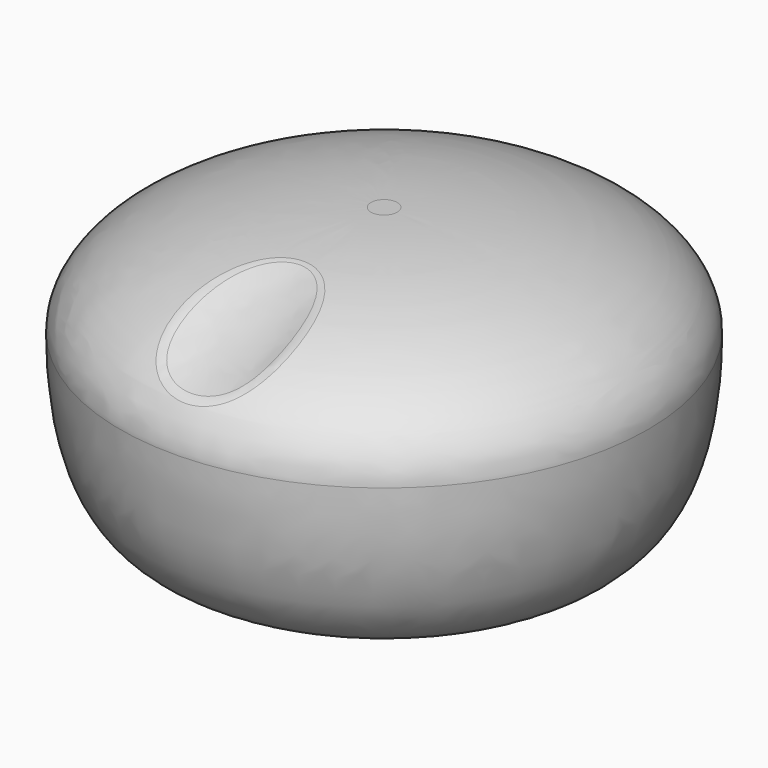
from build123d import *

# Parameters (mm, degrees)
F2_DEPTH  = 6.4135
F1_W      = 4.572
F1_H      = 1.397
F3_DEPTH  = 3.556
F5_W      = 5.5405606754
F5_H      = 2
F5_W_2    = 5.2343517082
F6_DEPTH  = 23
F7_W      = 1.3345703483
F7_H      = 2.6050336892
F10_DEPTH = 12.5
F5_W_3    = 2
F5_H_2    = 13.227
F11_DEPTH = 2
F5_W_4    = 12.4850876164
F12_DEPTH = 1
F13_DEPTH = 3.6
F17_DEPTH = 50
F18_R     = 3


with BuildPart() as f2:
    # F1 (on Front) → F2 (new body, symmetric)
    with BuildSketch(Plane.XZ):
        Polygon((-17.018, -11.176), (-17.018, -25.818), (5.842, -25.818), (5.842, -11.176), (10.668, -11.176), (10.668, -8.636), (5.842, -8.636), (5.842, 0), (2.286, 0), (-2.286, 0), (-5.842, 0), (-5.842, -4.318), (-17.018, -4.318), (-17.018, -8.636), (-22.098, -8.636), (-22.098, -11.176), align=None)
    extrude(amount=F2_DEPTH, both=True)

    # F1 (on Front) → F3 (join, symmetric)
    with BuildSketch(Plane.XZ):
        with Locations((0, 0.6985)):
            Rectangle(F1_W, F1_H)
        with Locations((0, 2.0955)):
            Rectangle(F1_W, F1_H)
    extrude(amount=F3_DEPTH, both=True)

    # F1 (on Front) → F13 (join, symmetric)
    with BuildSketch(Plane.XZ):
        Polygon((2.286, 2.794), (2.286, 1.397), (3.7302627534, 1.397), (3.7302627534, 3.882), (-3.4697372466, 3.882), (-3.4697372466, 1.397), (-2.286, 1.397), (-2.286, 2.794), align=None)
        Polygon((-3.4697372466, 3.882), (3.7302627534, 3.882), (3.7302627534, 5.482), (-14.9741563946, 5.482), (-14.9741563946, 3.882), align=None)
    extrude(amount=F13_DEPTH, both=True)


with BuildPart() as f4:
    # F0 (on Front) → F4 (revolve)
    with BuildSketch(Plane.XZ):
        with BuildLine():
            Line((24.9327979982, -23), (0, -23))
            Line((0, -23), (0, -26))
            Line((0, -26), (24.8083844781, -26))
            add(Edge.make_bspline(
                [(24.8083844781, -26), (35.2252668336, -26), (39.6886657653, -15.4061496672), (39.6886657653, 0)],
                knots=[0, 0, 0, 0, 29.9570153918, 29.9570153918, 29.9570153918, 29.9570153918], degree=3))
            Line((39.6886657653, 0), (38.1886657653, 0))
            Line((38.1886657653, 0), (38.1886657653, -3))
            Line((38.1886657653, -3), (36.6541846112, -3))
            add(Edge.make_bspline(
                [(24.9327979982, -23), (34.9615236875, -23), (36.4420685625, -10.8768821345), (36.6541846112, -3)],
                knots=[0, 0, 0, 0, 22.6723383484, 22.6723383484, 22.6723383484, 22.6723383484], degree=3))
        make_face()
    revolve(axis=Axis((0, 0, 12.485653162), (0, 0, 1)))

    # F5 (on face) → F6 (join, through all)
    with BuildSketch(Plane.XY.offset(-23)):
        with Locations((-14.4477196623, -7.6135)):
            Rectangle(F5_W, F5_H)
        with Locations((3.4248241459, -7.6135)):
            Rectangle(F5_W_2, F5_H)
        with Locations((3.4248241459, 7.6135)):
            Rectangle(F5_W_2, F5_H)
        with Locations((-14.4477196623, 7.6135)):
            Rectangle(F5_W, F5_H)
    extrude(amount=F6_DEPTH)

    # F5 (on face) → F11 (join)
    with BuildSketch(Plane.XY.offset(-23)):
        with Locations((7.042, 0)):
            Rectangle(F5_W_3, F5_H_2)
        with Locations((7.042, -7.6135)):
            Rectangle(F5_W_3, F5_H)
        with Locations((7.042, 7.6135)):
            Rectangle(F5_W_3, F5_H)
    extrude(amount=F11_DEPTH)

    # F5 (on face) → F12 (join)
    with BuildSketch(Plane.XY.offset(-23)):
        with Locations((-5.4348955164, -7.6135)):
            Rectangle(F5_W_4, F5_H)
        with Locations((-5.4348955164, 7.6135)):
            Rectangle(F5_W_4, F5_H)
        Polygon((-17.218, -8.6135), (-17.218, -6.6135), (-17.218, 6.6135), (-17.218, 8.6135), (-19.218, 8.6135), (-19.218, -8.6135), align=None)
    extrude(amount=F12_DEPTH)


with BuildPart() as f8:
    # F7 (on Front) → F8 (revolve)
    with BuildSketch(Plane.XZ):
        with BuildLine():
            Line((1.9791810773, 16.5), (0, 16.5))
            Line((0, 16.5), (0, 15))
            add(Edge.make_bspline(
                [(0, 15), (18.1219074875, 15), (36.6886657653, 9.8843509331), (36.6886657653, 0)],
                knots=[0, 0, 0, 0, 39.6365764873, 39.6365764873, 39.6365764873, 39.6365764873], degree=3))
            Line((36.6886657653, 0), (38.0232361135, 0))
            Line((38.0232361135, 0), (39.6886657653, 0))
            add(Edge.make_bspline(
                [(1.9791810773, 16.5), (22.9646191001, 16.5), (39.6886657653, 9.3534307705), (39.6886657653, 0)],
                knots=[0, 0, 0, 0, 41.1613317985, 41.1613317985, 41.1613317985, 41.1613317985], degree=3))
        make_face()
        with Locations((37.3559509394, -1.3025168446)):
            Rectangle(F7_W, F7_H)
    revolve(axis=Axis((0, 0, 12.485653162), (0, 0, 1)))

    # F9 (on Front) → F10 (join, symmetric)
    with BuildSketch(Plane.XZ):
        Polygon((-7.273943428, 3.9704855306), (-3.81, 3.9704855306), (-3.81, 13), (3.81, 13), (3.81, 3.9704855306), (7.273943428, 3.9704855306), (7.273943428, 15.2057409286), (-7.273943428, 15.2057409286), align=None)
    extrude(amount=F10_DEPTH, both=True)

    # F16 (on line) → F17 (cut)
    with BuildSketch(Plane(origin=(0, -41.3328305695, -17.5432446815), x_dir=(1, 0, 0), z_dir=(0, -0.9205168761, -0.3907028038))):
        with BuildLine():
            add(Edge.make_bspline(
                [(10, 23.7710124391), (10, 29.8331902656), (-5, 26.8021013524), (-20, 23.7710124391), (-5, 20.7399235259), (10, 17.7088346126), (10, 23.7710124391)],
                knots=[0, 0, 0, 2.0943951024, 2.0943951024, 4.1887902048, 4.1887902048, 6.2831853072, 6.2831853072, 6.2831853072], degree=2, weights=[1, 0.5, 1, 0.5, 1, 0.5, 1]))
        make_face()
    extrude(amount=-F17_DEPTH, mode=Mode.SUBTRACT)

    # F18
    f18_edges = [f8.edges().sort_by_distance(p)[0] for p in [
        (-7.331162, -23.271587, 13.360294),
    ]]
    fillet(f18_edges, radius=F18_R)


solid = Compound([f2.part, f4.part, f8.part])
